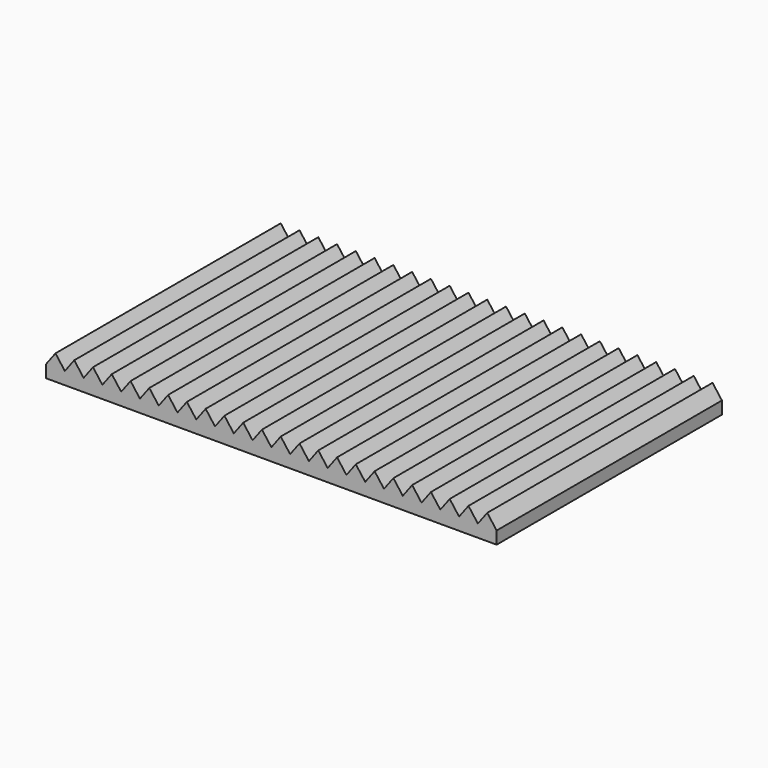
from build123d import *

# Parameters (mm, degrees)
F1_DEPTH = 254


# Not quite as in the source:
# - ends of sketch curves that miss each other by under 0.0002 mm in the source are joined


with BuildPart() as f1:
    # F0 (on Front) → F1 (new body)
    with BuildSketch(Plane.XZ):
        Polygon((-194.73333335, 16.9333332013), (-203.2, 5.6444444388), (-194.73333335, 5.6444444388), align=None)
        Polygon((-194.73333335, 5.6444444388), (-203.2, 5.6444444388), (-203.2, -5.6444444388), (203.2, -5.6444444388), (203.2, 5.6444444388), (186.26665915, 5.6444444388), (169.33332615, 5.6444444388), (152.39999315, 5.6444444388), (135.46666015, 5.6444444388), (118.53332715, 5.6444444388), (101.59999415, 5.6444444388), (84.66666115, 5.6444444388), (67.73332815, 5.6444444388), (50.79999515, 5.6444444388), (33.86666215, 5.6444444388), (16.93332915, 5.6444444388), (-3.85e-06, 5.6444444388), (-16.93333685, 5.6444444388), (-33.86666985, 5.6444444388), (-50.80000285, 5.6444444388), (-67.73333585, 5.6444444388), (-84.66666885, 5.6444444388), (-101.60000185, 5.6444444388), (-118.53333485, 5.6444444388), (-135.46666785, 5.6444444388), (-152.40000085, 5.6444444388), (-169.33333385, 5.6444444388), (-186.26666685, 5.6444444388), align=None)
        Polygon((-194.73333335, 16.9333332013), (-194.73333335, 5.6444444388), (-186.26666685, 5.6444444388), align=None)
        Polygon((-177.80000035, 16.9333332013), (-186.266667, 5.6444444388), (-169.33333385, 5.6444444388), align=None)
        Polygon((-160.86666735, 16.9333332013), (-169.333334, 5.6444444388), (-152.40000085, 5.6444444388), align=None)
        Polygon((186.26665915, 5.6444444388), (203.2, 5.6444444388), (194.73332565, 16.9333332013), align=None)
        Polygon((-143.93333435, 16.9333332013), (-152.400001, 5.6444444388), (-135.46666785, 5.6444444388), align=None)
        Polygon((169.33332615, 5.6444444388), (186.26665915, 5.6444444388), (177.79999265, 16.9333332013), align=None)
        Polygon((-127.00000135, 16.9333332013), (-135.466668, 5.6444444388), (-118.53333485, 5.6444444388), align=None)
        Polygon((152.39999315, 5.6444444388), (169.33332615, 5.6444444388), (160.86665965, 16.9333332013), align=None)
        Polygon((-110.06666835, 16.9333332013), (-118.533335, 5.6444444388), (-101.60000185, 5.6444444388), align=None)
        Polygon((135.46666015, 5.6444444388), (152.39999315, 5.6444444388), (143.93332665, 16.9333332013), align=None)
        Polygon((-93.13333535, 16.9333332013), (-101.600002, 5.6444444388), (-84.66666885, 5.6444444388), align=None)
        Polygon((118.53332715, 5.6444444388), (135.46666015, 5.6444444388), (126.99999365, 16.9333332013), align=None)
        Polygon((-76.20000235, 16.9333332013), (-84.666669, 5.6444444388), (-67.73333585, 5.6444444388), align=None)
        Polygon((101.59999415, 5.6444444388), (118.53332715, 5.6444444388), (110.06666065, 16.9333332013), align=None)
        Polygon((-59.26666935, 16.9333332013), (-67.733336, 5.6444444388), (-50.80000285, 5.6444444388), align=None)
        Polygon((84.66666115, 5.6444444388), (101.59999415, 5.6444444388), (93.13332765, 16.9333332013), align=None)
        Polygon((-42.33333635, 16.9333332013), (-50.800003, 5.6444444388), (-33.86666985, 5.6444444388), align=None)
        Polygon((67.73332815, 5.6444444388), (84.66666115, 5.6444444388), (76.19999465, 16.9333332013), align=None)
        Polygon((-25.40000335, 16.9333332013), (-33.86667, 5.6444444388), (-16.93333685, 5.6444444388), align=None)
        Polygon((50.79999515, 5.6444444388), (67.73332815, 5.6444444388), (59.26666165, 16.9333332013), align=None)
        Polygon((-8.46667035, 16.9333332013), (-16.933337, 5.6444444388), (-3.85e-06, 5.6444444388), align=None)
        Polygon((33.86666215, 5.6444444388), (50.79999515, 5.6444444388), (42.33332865, 16.9333332013), align=None)
        Polygon((8.46666265, 16.9333332013), (-4e-06, 5.6444444388), (16.93332915, 5.6444444388), align=None)
        Polygon((16.93332915, 5.6444444388), (33.86666215, 5.6444444388), (25.39999565, 16.9333332013), align=None)
    extrude(amount=F1_DEPTH)


solid = f1.part
